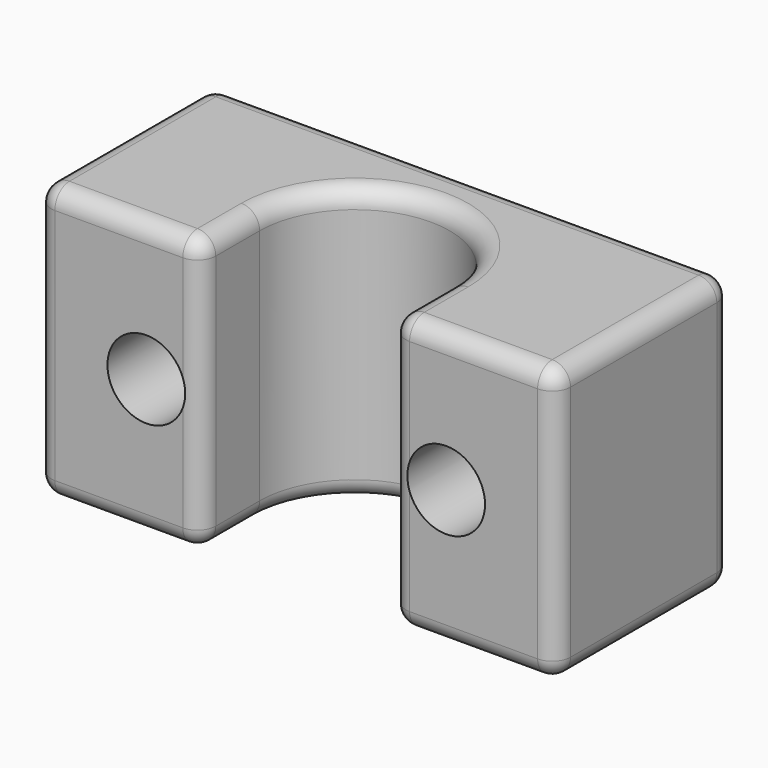
from build123d import *

# Parameters (mm, degrees)
F1_DEPTH     = 15
F2_R         = 2.125
F3_DEPTH     = 12.001
F4_T1_DEPTH  = 3
F4_T3_DEPTH  = 7
F4_T5_DEPTH  = 10
F4_T7_DEPTH  = 26.4
F4_T9_DEPTH  = 7
F4_T11_DEPTH = 13
F4_S15_W     = 1
F4_S15_H     = 1
F4_T16_DEPTH = 1
F4_S21_W     = 1
F4_S21_H     = 1
F4_T22_DEPTH = 1
F4_S27_W     = 1
F4_S27_H     = 1
F4_T28_DEPTH = 1
F4_S33_W     = 1
F4_S33_H     = 1
F4_T34_DEPTH = 1
F4_S39_W     = 1
F4_S39_H     = 1
F4_T40_DEPTH = 1
F4_S45_W     = 1
F4_S45_H     = 1
F4_T46_DEPTH = 1
F4_S51_W     = 1
F4_S51_H     = 1
F4_T52_DEPTH = 1
F4_S57_W     = 1
F4_S57_H     = 1
F4_T58_DEPTH = 1
F4_S63_W     = 1
F4_S63_H     = 1
F4_T64_DEPTH = 1
F4_S69_W     = 1
F4_S69_H     = 1
F4_T70_DEPTH = 1
F4_S75_W     = 1
F4_S75_H     = 1
F4_T76_DEPTH = 1
F4_S81_W     = 1
F4_S81_H     = 1
F4_T82_DEPTH = 1
F4_T86_ANGLE = 180
F4_T88_ANGLE = 180


# Not quite as in the source:
# - a fillet or chamfer that OpenCascade refuses, or shapes differently, is made with other operations: its cross-section is extruded or revolved along the edge and cut away or added


with BuildPart() as f1:
    # F0 (on Top) → F1 (new body)
    with BuildSketch(Plane.XY):
        with BuildLine():
            Line((5.2, 4), (5.2, 0))
            Line((5.2, 0), (14.2, 0))
            Line((14.2, 0), (14.2, 12))
            Line((14.2, 12), (-14.2, 12))
            Line((-14.2, 12), (-14.2, 0))
            Line((-14.2, 0), (-5.2, 0))
            Line((-5.2, 0), (-5.2, 4))
            ThreePointArc((-5.2, 4), (0, 9.2), (5.2, 4))
        make_face()
    extrude(amount=F1_DEPTH)

    # F2 (on face) → F3 (cut, through all)
    with BuildSketch(Plane.XZ):
        with Locations((-8.2, 7.5)):
            Circle(F2_R)
        with Locations((8.2, 7.5)):
            Circle(F2_R)
    extrude(amount=-F3_DEPTH, mode=Mode.SUBTRACT)

    # F4: fillet of radius 1 on 22 edges, made by hand

    # F4_s2 → F4_t1 (cut)
    with BuildSketch(Plane.XZ.offset(-4)):
        with BuildLine():
            ThreePointArc((-5.2, 14), (-5.4928932188, 14.7071067812), (-6.2, 15))
            Line((-6.2, 15), (-5.2, 15))
            Line((-5.2, 15), (-5.2, 14))
        make_face()
        with BuildLine():
            ThreePointArc((6.2, 15), (5.4928932188, 14.7071067812), (5.2, 14))
            Line((5.2, 14), (5.2, 15))
            Line((5.2, 15), (6.2, 15))
        make_face()
        with BuildLine():
            ThreePointArc((-5.2, 1), (-5.4928932188, 0.2928932188), (-6.2, 0))
            Line((-6.2, 0), (-5.2, 0))
            Line((-5.2, 0), (-5.2, 1))
        make_face()
        with BuildLine():
            ThreePointArc((6.2, 0), (5.4928932188, 0.2928932188), (5.2, 1))
            Line((5.2, 1), (5.2, 0))
            Line((5.2, 0), (6.2, 0))
        make_face()
    extrude(amount=F4_T1_DEPTH, mode=Mode.SUBTRACT)

    # F4_s4 → F4_t3 (cut)
    with BuildSketch(Plane.YZ.offset(6.2)):
        with BuildLine():
            ThreePointArc((1, 15), (0.2928932188, 14.7071067812), (0, 14))
            Line((0, 14), (0, 15))
            Line((0, 15), (1, 15))
        make_face()
        with BuildLine():
            ThreePointArc((1, 0), (0.2928932188, 0.2928932188), (0, 1))
            Line((0, 1), (0, 0))
            Line((0, 0), (1, 0))
        make_face()
    extrude(amount=F4_T3_DEPTH, mode=Mode.SUBTRACT)

    # F4_s6 → F4_t5 (cut)
    with BuildSketch(Plane.XZ.offset(-11)):
        with BuildLine():
            ThreePointArc((13.2, 15), (13.9071067812, 14.7071067812), (14.2, 14))
            Line((14.2, 14), (14.2, 15))
            Line((14.2, 15), (13.2, 15))
        make_face()
        with BuildLine():
            ThreePointArc((-13.2, 15), (-13.9071067812, 14.7071067812), (-14.2, 14))
            Line((-14.2, 14), (-14.2, 15))
            Line((-14.2, 15), (-13.2, 15))
        make_face()
        with BuildLine():
            ThreePointArc((-13.2, 0), (-13.9071067812, 0.2928932188), (-14.2, 1))
            Line((-14.2, 1), (-14.2, 0))
            Line((-14.2, 0), (-13.2, 0))
        make_face()
        with BuildLine():
            ThreePointArc((13.2, 0), (13.9071067812, 0.2928932188), (14.2, 1))
            Line((14.2, 1), (14.2, 0))
            Line((14.2, 0), (13.2, 0))
        make_face()
    extrude(amount=F4_T5_DEPTH, mode=Mode.SUBTRACT)

    # F4_s8 → F4_t7 (cut)
    with BuildSketch(Plane.YZ.offset(-13.2)):
        with BuildLine():
            ThreePointArc((11, 15), (11.7071067812, 14.7071067812), (12, 14))
            Line((12, 14), (12, 15))
            Line((12, 15), (11, 15))
        make_face()
        with BuildLine():
            ThreePointArc((11, 0), (11.7071067812, 0.2928932188), (12, 1))
            Line((12, 1), (12, 0))
            Line((12, 0), (11, 0))
        make_face()
    extrude(amount=F4_T7_DEPTH, mode=Mode.SUBTRACT)

    # F4_s10 → F4_t9 (cut)
    with BuildSketch(Plane.YZ.offset(-13.2)):
        with BuildLine():
            ThreePointArc((0, 14), (0.2928932188, 14.7071067812), (1, 15))
            Line((1, 15), (0, 15))
            Line((0, 15), (0, 14))
        make_face()
        with BuildLine():
            ThreePointArc((0, 1), (0.2928932188, 0.2928932188), (1, 0))
            Line((1, 0), (0, 0))
            Line((0, 0), (0, 1))
        make_face()
    extrude(amount=F4_T9_DEPTH, mode=Mode.SUBTRACT)

    # F4_s12 → F4_t11 (cut)
    with BuildSketch(Plane.XY.offset(1)):
        with BuildLine():
            ThreePointArc((-14.2, 11), (-13.9071067812, 11.7071067812), (-13.2, 12))
            Line((-13.2, 12), (-14.2, 12))
            Line((-14.2, 12), (-14.2, 11))
        make_face()
        with BuildLine():
            ThreePointArc((-13.2, 0), (-13.9071067812, 0.2928932188), (-14.2, 1))
            Line((-14.2, 1), (-14.2, 0))
            Line((-14.2, 0), (-13.2, 0))
        make_face()
        with BuildLine():
            ThreePointArc((13.2, 0), (13.9071067812, 0.2928932188), (14.2, 1))
            Line((14.2, 1), (14.2, 0))
            Line((14.2, 0), (13.2, 0))
        make_face()
        with BuildLine():
            ThreePointArc((14.2, 11), (13.9071067812, 11.7071067812), (13.2, 12))
            Line((13.2, 12), (14.2, 12))
            Line((14.2, 12), (14.2, 11))
        make_face()
        with BuildLine():
            ThreePointArc((-5.2, 1), (-5.4928932188, 0.2928932188), (-6.2, 0))
            Line((-6.2, 0), (-5.2, 0))
            Line((-5.2, 0), (-5.2, 1))
        make_face()
        with BuildLine():
            ThreePointArc((5.2, 1), (5.4928932188, 0.2928932188), (6.2, 0))
            Line((6.2, 0), (5.2, 0))
            Line((5.2, 0), (5.2, 1))
        make_face()
    extrude(amount=F4_T11_DEPTH, mode=Mode.SUBTRACT)


with BuildPart() as f4_tool14:
    # F4_s15 → F4_t16 (new body)
    with BuildSketch(Plane.YZ.offset(-6.2)):
        with Locations((0.5, 14.5)):
            Rectangle(F4_S15_W, F4_S15_H)
    extrude(amount=F4_T16_DEPTH)

    # F4_s17 → F4_t18 (revolve, cut)
    with BuildSketch(Plane(origin=(-6.2, 1, 14), x_dir=(0, 0.7071067812, -0.7071067812), z_dir=(0, -0.7071067812, -0.7071067812))):
        with BuildLine():
            ThreePointArc((0, -1), (1, 0), (0, 1))
            Line((0, 1), (0, -1))
        make_face()
    revolve(axis=Axis((-6.2, 1, 14), (1, 0, 0)), mode=Mode.SUBTRACT)


with BuildPart() as f1_1:
    add(f1.part)

    # F4_t13: cut F4_tool14
    add(f4_tool14.part, mode=Mode.SUBTRACT)


with BuildPart() as f4_tool20:
    # F4_s21 → F4_t22 (new body)
    with BuildSketch(Plane.XZ.offset(-1)):
        with Locations((5.7, 14.5)):
            Rectangle(F4_S21_W, F4_S21_H)
    extrude(amount=F4_T22_DEPTH)

    # F4_s23 → F4_t24 (revolve, cut)
    with BuildSketch(Plane(origin=(6.2, 1, 14), x_dir=(0.7071067812, 0, -0.7071067812), z_dir=(-0.7071067812, 0, -0.7071067812))):
        with BuildLine():
            ThreePointArc((0, -1), (1, 0), (0, 1))
            Line((0, 1), (0, -1))
        make_face()
    revolve(axis=Axis((6.2, 1, 14), (0, -1, 0)), mode=Mode.SUBTRACT)


with BuildPart() as f1_2:
    add(f1_1.part)

    # F4_t19: cut F4_tool20
    add(f4_tool20.part, mode=Mode.SUBTRACT)


with BuildPart() as f4_tool26:
    # F4_s27 → F4_t28 (new body)
    with BuildSketch(Plane.XZ.offset(-1)):
        with Locations((13.7, 14.5)):
            Rectangle(F4_S27_W, F4_S27_H)
    extrude(amount=F4_T28_DEPTH)

    # F4_s29 → F4_t30 (revolve, cut)
    with BuildSketch(Plane(origin=(13.2, 1, 14), x_dir=(-0.7071067812, 0, -0.7071067812), z_dir=(-0.7071067812, 0, 0.7071067812))):
        with BuildLine():
            ThreePointArc((0, -1), (1, 0), (0, 1))
            Line((0, 1), (0, -1))
        make_face()
    revolve(axis=Axis((13.2, 1, 14), (0, -1, 0)), mode=Mode.SUBTRACT)


with BuildPart() as f1_3:
    add(f1_2.part)

    # F4_t25: cut F4_tool26
    add(f4_tool26.part, mode=Mode.SUBTRACT)


with BuildPart() as f4_tool32:
    # F4_s33 → F4_t34 (new body)
    with BuildSketch(Plane.YZ.offset(13.2)):
        with Locations((11.5, 14.5)):
            Rectangle(F4_S33_W, F4_S33_H)
    extrude(amount=F4_T34_DEPTH)

    # F4_s35 → F4_t36 (revolve, cut)
    with BuildSketch(Plane(origin=(13.2, 11, 14), x_dir=(0, -0.7071067812, -0.7071067812), z_dir=(0, -0.7071067812, 0.7071067812))):
        with BuildLine():
            ThreePointArc((0, -1), (1, 0), (0, 1))
            Line((0, 1), (0, -1))
        make_face()
    revolve(axis=Axis((13.2, 11, 14), (1, 0, 0)), mode=Mode.SUBTRACT)


with BuildPart() as f1_4:
    add(f1_3.part)

    # F4_t31: cut F4_tool32
    add(f4_tool32.part, mode=Mode.SUBTRACT)


with BuildPart() as f4_tool38:
    # F4_s39 → F4_t40 (new body)
    with BuildSketch(Plane.XZ.offset(-11)):
        with Locations((-13.7, 14.5)):
            Rectangle(F4_S39_W, F4_S39_H)
    extrude(amount=-F4_T40_DEPTH)

    # F4_s41 → F4_t42 (revolve, cut)
    with BuildSketch(Plane(origin=(-13.2, 11, 14), x_dir=(0.7071067812, 0, -0.7071067812), z_dir=(0.7071067812, 0, 0.7071067812))):
        with BuildLine():
            ThreePointArc((0, -1), (1, 0), (0, 1))
            Line((0, 1), (0, -1))
        make_face()
    revolve(axis=Axis((-13.2, 11, 14), (0, 1, 0)), mode=Mode.SUBTRACT)


with BuildPart() as f1_5:
    add(f1_4.part)

    # F4_t37: cut F4_tool38
    add(f4_tool38.part, mode=Mode.SUBTRACT)


with BuildPart() as f4_tool44:
    # F4_s45 → F4_t46 (new body)
    with BuildSketch(Plane.XZ.offset(-1)):
        with Locations((-13.7, 14.5)):
            Rectangle(F4_S45_W, F4_S45_H)
    extrude(amount=F4_T46_DEPTH)

    # F4_s47 → F4_t48 (revolve, cut)
    with BuildSketch(Plane(origin=(-13.2, 1, 14), x_dir=(0.7071067812, 0, -0.7071067812), z_dir=(-0.7071067812, 0, -0.7071067812))):
        with BuildLine():
            ThreePointArc((0, -1), (1, 0), (0, 1))
            Line((0, 1), (0, -1))
        make_face()
    revolve(axis=Axis((-13.2, 1, 14), (0, -1, 0)), mode=Mode.SUBTRACT)


with BuildPart() as f1_6:
    add(f1_5.part)

    # F4_t43: cut F4_tool44
    add(f4_tool44.part, mode=Mode.SUBTRACT)


with BuildPart() as f4_tool50:
    # F4_s51 → F4_t52 (new body)
    with BuildSketch(Plane.XZ.offset(-11)):
        with Locations((-13.7, 0.5)):
            Rectangle(F4_S51_W, F4_S51_H)
    extrude(amount=-F4_T52_DEPTH)

    # F4_s53 → F4_t54 (revolve, cut)
    with BuildSketch(Plane(origin=(-13.2, 11, 1), x_dir=(0.7071067812, 0, 0.7071067812), z_dir=(-0.7071067812, 0, 0.7071067812))):
        with BuildLine():
            ThreePointArc((0, -1), (1, 0), (0, 1))
            Line((0, 1), (0, -1))
        make_face()
    revolve(axis=Axis((-13.2, 11, 1), (0, 1, 0)), mode=Mode.SUBTRACT)


with BuildPart() as f1_7:
    add(f1_6.part)

    # F4_t49: cut F4_tool50
    add(f4_tool50.part, mode=Mode.SUBTRACT)


with BuildPart() as f4_tool56:
    # F4_s57 → F4_t58 (new body)
    with BuildSketch(Plane.XZ.offset(-1)):
        with Locations((-13.7, 0.5)):
            Rectangle(F4_S57_W, F4_S57_H)
    extrude(amount=F4_T58_DEPTH)

    # F4_s59 → F4_t60 (revolve, cut)
    with BuildSketch(Plane(origin=(-13.2, 1, 1), x_dir=(0.7071067812, 0, 0.7071067812), z_dir=(0.7071067812, 0, -0.7071067812))):
        with BuildLine():
            ThreePointArc((0, -1), (1, 0), (0, 1))
            Line((0, 1), (0, -1))
        make_face()
    revolve(axis=Axis((-13.2, 1, 1), (0, -1, 0)), mode=Mode.SUBTRACT)


with BuildPart() as f1_8:
    add(f1_7.part)

    # F4_t55: cut F4_tool56
    add(f4_tool56.part, mode=Mode.SUBTRACT)


with BuildPart() as f4_tool62:
    # F4_s63 → F4_t64 (new body)
    with BuildSketch(Plane.YZ.offset(-6.2)):
        with Locations((0.5, 0.5)):
            Rectangle(F4_S63_W, F4_S63_H)
    extrude(amount=F4_T64_DEPTH)

    # F4_s65 → F4_t66 (revolve, cut)
    with BuildSketch(Plane(origin=(-6.2, 1, 1), x_dir=(0, 0.7071067812, 0.7071067812), z_dir=(0, 0.7071067812, -0.7071067812))):
        with BuildLine():
            ThreePointArc((0, -1), (1, 0), (0, 1))
            Line((0, 1), (0, -1))
        make_face()
    revolve(axis=Axis((-6.2, 1, 1), (1, 0, 0)), mode=Mode.SUBTRACT)


with BuildPart() as f1_9:
    add(f1_8.part)

    # F4_t61: cut F4_tool62
    add(f4_tool62.part, mode=Mode.SUBTRACT)


with BuildPart() as f4_tool68:
    # F4_s69 → F4_t70 (new body)
    with BuildSketch(Plane.XZ.offset(-1)):
        with Locations((5.7, 0.5)):
            Rectangle(F4_S69_W, F4_S69_H)
    extrude(amount=F4_T70_DEPTH)

    # F4_s71 → F4_t72 (revolve, cut)
    with BuildSketch(Plane(origin=(6.2, 1, 1), x_dir=(0.7071067812, 0, 0.7071067812), z_dir=(0.7071067812, 0, -0.7071067812))):
        with BuildLine():
            ThreePointArc((0, -1), (1, 0), (0, 1))
            Line((0, 1), (0, -1))
        make_face()
    revolve(axis=Axis((6.2, 1, 1), (0, -1, 0)), mode=Mode.SUBTRACT)


with BuildPart() as f1_10:
    add(f1_9.part)

    # F4_t67: cut F4_tool68
    add(f4_tool68.part, mode=Mode.SUBTRACT)


with BuildPart() as f4_tool74:
    # F4_s75 → F4_t76 (new body)
    with BuildSketch(Plane.XZ.offset(-1)):
        with Locations((13.7, 0.5)):
            Rectangle(F4_S75_W, F4_S75_H)
    extrude(amount=F4_T76_DEPTH)

    # F4_s77 → F4_t78 (revolve, cut)
    with BuildSketch(Plane(origin=(13.2, 1, 1), x_dir=(-0.7071067812, 0, 0.7071067812), z_dir=(0.7071067812, 0, 0.7071067812))):
        with BuildLine():
            ThreePointArc((0, -1), (1, 0), (0, 1))
            Line((0, 1), (0, -1))
        make_face()
    revolve(axis=Axis((13.2, 1, 1), (0, -1, 0)), mode=Mode.SUBTRACT)


with BuildPart() as f1_11:
    add(f1_10.part)

    # F4_t73: cut F4_tool74
    add(f4_tool74.part, mode=Mode.SUBTRACT)


with BuildPart() as f4_tool80:
    # F4_s81 → F4_t82 (new body)
    with BuildSketch(Plane.YZ.offset(13.2)):
        with Locations((11.5, 0.5)):
            Rectangle(F4_S81_W, F4_S81_H)
    extrude(amount=F4_T82_DEPTH)

    # F4_s83 → F4_t84 (revolve, cut)
    with BuildSketch(Plane(origin=(13.2, 11, 1), x_dir=(0, -0.7071067812, 0.7071067812), z_dir=(0, 0.7071067812, 0.7071067812))):
        with BuildLine():
            ThreePointArc((0, -1), (1, 0), (0, 1))
            Line((0, 1), (0, -1))
        make_face()
    revolve(axis=Axis((13.2, 11, 1), (1, 0, 0)), mode=Mode.SUBTRACT)


with BuildPart() as f1_12:
    add(f1_11.part)

    # F4_t79: cut F4_tool80
    add(f4_tool80.part, mode=Mode.SUBTRACT)

    # F4_s85 → F4_t86 (revolve, cut)
    with BuildSketch(Plane.XZ.offset(-4)):
        with BuildLine():
            ThreePointArc((-5.2, 14), (-5.4928932188, 14.7071067812), (-6.2, 15))
            Line((-6.2, 15), (-5.2, 15))
            Line((-5.2, 15), (-5.2, 14))
        make_face()
    revolve(axis=Axis((0, 4, 15), (0, 0, -1)), revolution_arc=F4_T86_ANGLE, mode=Mode.SUBTRACT)

    # F4_s87 → F4_t88 (revolve, cut)
    with BuildSketch(Plane.XZ.offset(-4)):
        with BuildLine():
            ThreePointArc((-5.2, 1), (-5.4928932188, 0.2928932188), (-6.2, 0))
            Line((-6.2, 0), (-5.2, 0))
            Line((-5.2, 0), (-5.2, 1))
        make_face()
    revolve(axis=Axis((0, 4, 0), (0, 0, -1)), revolution_arc=F4_T88_ANGLE, mode=Mode.SUBTRACT)


solid = f1_12.part
